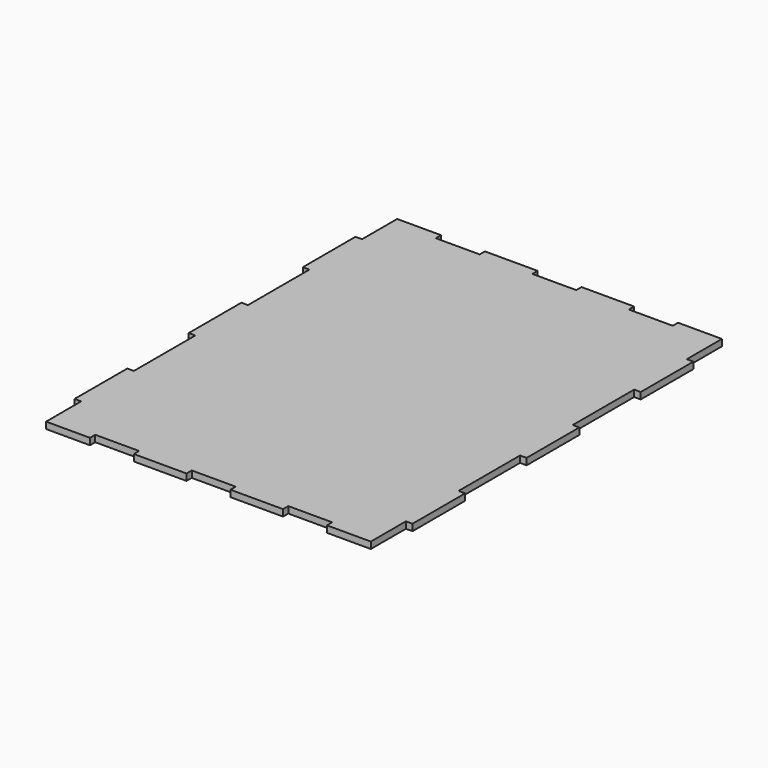
from build123d import *

# Parameters (mm, degrees)
F1_DEPTH = 3
F2_W     = 20
F2_H     = 3
F3_DEPTH = 3.001


# Not quite as in the source:
# - a feature names something its author has since deleted; it is built from what else it names


with BuildPart() as f1:
    # F0 (on Top) → F1 (new body)
    with BuildSketch(Plane.XY):
        Polygon((-74, 0), (0, 0), (74, 0), (74, 20), (77, 20), (77, 50), (74, 50), (74, 85), (77, 85), (77, 115), (74, 115), (74, 150), (77, 150), (77, 180), (74, 180), (74, 200), (0, 200), (-74, 200), (-74, 180), (-77, 180), (-77, 150), (-74, 150), (-74, 115), (-77, 115), (-77, 85), (-74, 85), (-74, 50), (-77, 50), (-77, 20), (-74, 20), align=None)
    extrude(amount=F1_DEPTH)

    # F2 (on face) → F3 (cut, through all)
    with BuildSketch(Plane.XY.offset(3)):
        with Locations((-44, 1.5)):
            Rectangle(F2_W, F2_H)
        with Locations((44, 1.5)):
            Rectangle(F2_W, F2_H)
        with Locations((0, 1.5)):
            Rectangle(F2_W, F2_H)
        with Locations((-44, 198.5)):
            Rectangle(F2_W, F2_H)
        with Locations((44, 198.5)):
            Rectangle(F2_W, F2_H)
        with Locations((0, 198.5)):
            Rectangle(F2_W, F2_H)
    extrude(amount=-F3_DEPTH, mode=Mode.SUBTRACT)


solid = f1.part
